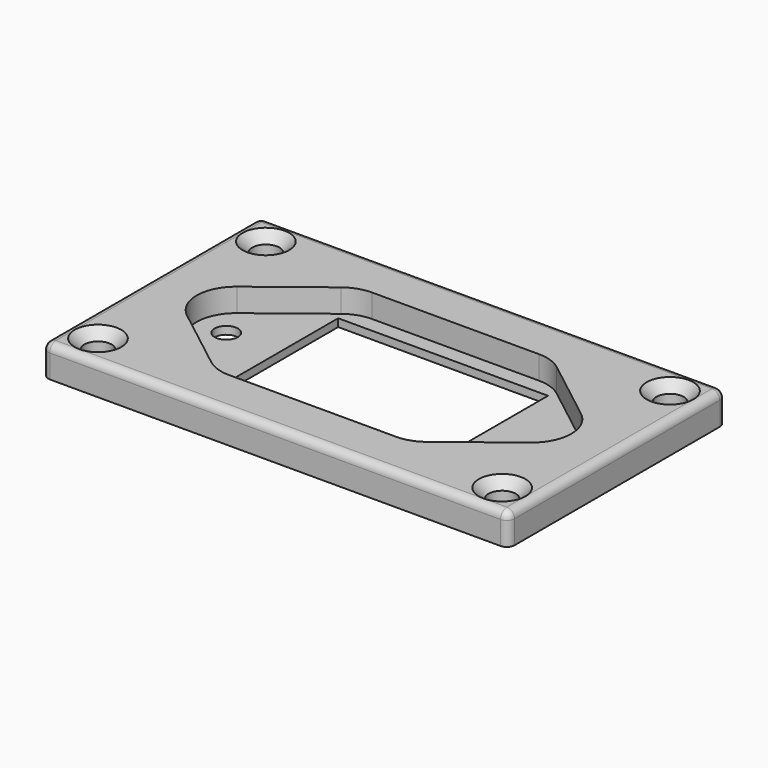
from build123d import *

# Parameters (mm, degrees)
F0_W           = 60
F0_H           = 35
F1_DEPTH       = 4
F3_DEPTH       = 3
F4_R           = 5.08
F5_W           = 27
F5_H           = 19
F6_DEPTH       = 25.4
F8_D           = 3.5
F8_CSINK_D     = 6
F8_CSINK_ANGLE = 90
F9_D           = 3
F10_T1_DEPTH   = 58
F10_T3_DEPTH   = 33
F10_T5_DEPTH   = 5.5
F10_S9_W       = 1
F10_S9_H       = 1
F10_T10_DEPTH  = 1
F10_S15_W      = 1
F10_S15_H      = 1
F10_T16_DEPTH  = 1
F10_S21_W      = 1
F10_S21_H      = 1
F10_T22_DEPTH  = 1
F10_S27_W      = 1
F10_S27_H      = 1
F10_T28_DEPTH  = 1


# Not quite as in the source:
# - a fillet or chamfer that OpenCascade refuses, or shapes differently, is made with other operations: its cross-section is extruded or revolved along the edge and cut away or added


with BuildPart() as f1:
    # F0 (on Top) → F1 (new body)
    with BuildSketch(Plane.XY):
        Rectangle(F0_W, F0_H)
    extrude(amount=F1_DEPTH)

    # F2 (on face) → F3 (cut)
    with BuildSketch(Plane.XY.offset(4)):
        Polygon((-27.3, 0), (-12.5, -11.5), (12.5, -11.5), (27.3, 0), (12.5, 11.5), (-12.5, 11.5), align=None)
    extrude(amount=-F3_DEPTH, mode=Mode.SUBTRACT)

    # F4
    f4_edges = [f1.edges().sort_by_distance(p)[0] for p in [
        (12.5, 11.5, 2.5),
        (12.5, -11.5, 2.5),
        (-12.5, -11.5, 2.5),
        (-12.5, 11.5, 2.5),
        (27.3, 0, 2.5),
        (-27.3, 0, 2.5),
    ]]
    fillet(f4_edges, radius=F4_R)

    # F5 (on face) → F6 (cut)
    with BuildSketch(Plane.XY.offset(1)):
        Rectangle(F5_W, F5_H)
    extrude(amount=-F6_DEPTH, mode=Mode.SUBTRACT)

    # F8 (through all)
    with Locations(Plane.XY.offset(4)):
        with Locations((-26, 13.5), (26, 13.5), (26, -13.5), (-26, -13.5)):
            CounterSinkHole(F8_D / 2, F8_CSINK_D / 2, counter_sink_angle=F8_CSINK_ANGLE)

    # F9 (through all)
    with Locations(Plane.XY.offset(4)):
        with Locations((-20.3, 0), (20.3, 0)):
            Hole(F9_D / 2)

    # F10: fillet of radius 1 on 8 edges, made by hand

    # F10_s2 → F10_t1 (cut)
    with BuildSketch(Plane.YZ.offset(-29)):
        with BuildLine():
            ThreePointArc((16.5, 4), (17.2071067812, 3.7071067812), (17.5, 3))
            Line((17.5, 3), (17.5, 4))
            Line((17.5, 4), (16.5, 4))
        make_face()
        with BuildLine():
            ThreePointArc((-16.5, 4), (-17.2071067812, 3.7071067812), (-17.5, 3))
            Line((-17.5, 3), (-17.5, 4))
            Line((-17.5, 4), (-16.5, 4))
        make_face()
    extrude(amount=F10_T1_DEPTH, mode=Mode.SUBTRACT)

    # F10_s4 → F10_t3 (cut)
    with BuildSketch(Plane.XZ.offset(-16.5)):
        with BuildLine():
            ThreePointArc((-29, 4), (-29.7071067812, 3.7071067812), (-30, 3))
            Line((-30, 3), (-30, 4))
            Line((-30, 4), (-29, 4))
        make_face()
        with BuildLine():
            ThreePointArc((29, 4), (29.7071067812, 3.7071067812), (30, 3))
            Line((30, 3), (30, 4))
            Line((30, 4), (29, 4))
        make_face()
    extrude(amount=F10_T3_DEPTH, mode=Mode.SUBTRACT)

    # F10_s6 → F10_t5 (cut)
    with BuildSketch(Plane.XY.offset(-2.5)):
        with BuildLine():
            ThreePointArc((30, -16.5), (29.7071067812, -17.2071067812), (29, -17.5))
            Line((29, -17.5), (30, -17.5))
            Line((30, -17.5), (30, -16.5))
        make_face()
        with BuildLine():
            ThreePointArc((29, 17.5), (29.7071067812, 17.2071067812), (30, 16.5))
            Line((30, 16.5), (30, 17.5))
            Line((30, 17.5), (29, 17.5))
        make_face()
        with BuildLine():
            ThreePointArc((-30, -16.5), (-29.7071067812, -17.2071067812), (-29, -17.5))
            Line((-29, -17.5), (-30, -17.5))
            Line((-30, -17.5), (-30, -16.5))
        make_face()
        with BuildLine():
            ThreePointArc((-29, 17.5), (-29.7071067812, 17.2071067812), (-30, 16.5))
            Line((-30, 16.5), (-30, 17.5))
            Line((-30, 17.5), (-29, 17.5))
        make_face()
    extrude(amount=F10_T5_DEPTH, mode=Mode.SUBTRACT)


with BuildPart() as f10_tool8:
    # F10_s9 → F10_t10 (new body)
    with BuildSketch(Plane.XY.offset(3)):
        with Locations((29.5, 17)):
            Rectangle(F10_S9_W, F10_S9_H)
    extrude(amount=F10_T10_DEPTH)

    # F10_s11 → F10_t12 (revolve, cut)
    with BuildSketch(Plane(origin=(29, 16.5, 3), x_dir=(-0.7071067812, -0.7071067812, 0), z_dir=(-0.7071067812, 0.7071067812, 0))):
        with BuildLine():
            ThreePointArc((0, -1), (1, 0), (0, 1))
            Line((0, 1), (0, -1))
        make_face()
    revolve(axis=Axis((29, 16.5, 3), (0, 0, 1)), mode=Mode.SUBTRACT)


with BuildPart() as f1_1:
    add(f1.part)

    # F10_t7: cut F10_tool8
    add(f10_tool8.part, mode=Mode.SUBTRACT)


with BuildPart() as f10_tool14:
    # F10_s15 → F10_t16 (new body)
    with BuildSketch(Plane.XY.offset(3)):
        with Locations((-29.5, 17)):
            Rectangle(F10_S15_W, F10_S15_H)
    extrude(amount=F10_T16_DEPTH)

    # F10_s17 → F10_t18 (revolve, cut)
    with BuildSketch(Plane(origin=(-29, 16.5, 3), x_dir=(0.7071067812, -0.7071067812, 0), z_dir=(-0.7071067812, -0.7071067812, 0))):
        with BuildLine():
            ThreePointArc((0, -1), (1, 0), (0, 1))
            Line((0, 1), (0, -1))
        make_face()
    revolve(axis=Axis((-29, 16.5, 3), (0, 0, 1)), mode=Mode.SUBTRACT)


with BuildPart() as f1_2:
    add(f1_1.part)

    # F10_t13: cut F10_tool14
    add(f10_tool14.part, mode=Mode.SUBTRACT)


with BuildPart() as f10_tool20:
    # F10_s21 → F10_t22 (new body)
    with BuildSketch(Plane.XY.offset(3)):
        with Locations((-29.5, -17)):
            Rectangle(F10_S21_W, F10_S21_H)
    extrude(amount=F10_T22_DEPTH)

    # F10_s23 → F10_t24 (revolve, cut)
    with BuildSketch(Plane(origin=(-29, -16.5, 3), x_dir=(0.7071067812, 0.7071067812, 0), z_dir=(0.7071067812, -0.7071067812, 0))):
        with BuildLine():
            ThreePointArc((0, -1), (1, 0), (0, 1))
            Line((0, 1), (0, -1))
        make_face()
    revolve(axis=Axis((-29, -16.5, 3), (0, 0, 1)), mode=Mode.SUBTRACT)


with BuildPart() as f1_3:
    add(f1_2.part)

    # F10_t19: cut F10_tool20
    add(f10_tool20.part, mode=Mode.SUBTRACT)


with BuildPart() as f10_tool26:
    # F10_s27 → F10_t28 (new body)
    with BuildSketch(Plane.XY.offset(3)):
        with Locations((29.5, -17)):
            Rectangle(F10_S27_W, F10_S27_H)
    extrude(amount=F10_T28_DEPTH)

    # F10_s29 → F10_t30 (revolve, cut)
    with BuildSketch(Plane(origin=(29, -16.5, 3), x_dir=(-0.7071067812, 0.7071067812, 0), z_dir=(0.7071067812, 0.7071067812, 0))):
        with BuildLine():
            ThreePointArc((0, -1), (1, 0), (0, 1))
            Line((0, 1), (0, -1))
        make_face()
    revolve(axis=Axis((29, -16.5, 3), (0, 0, 1)), mode=Mode.SUBTRACT)


with BuildPart() as f1_4:
    add(f1_3.part)

    # F10_t25: cut F10_tool26
    add(f10_tool26.part, mode=Mode.SUBTRACT)


solid = f1_4.part
